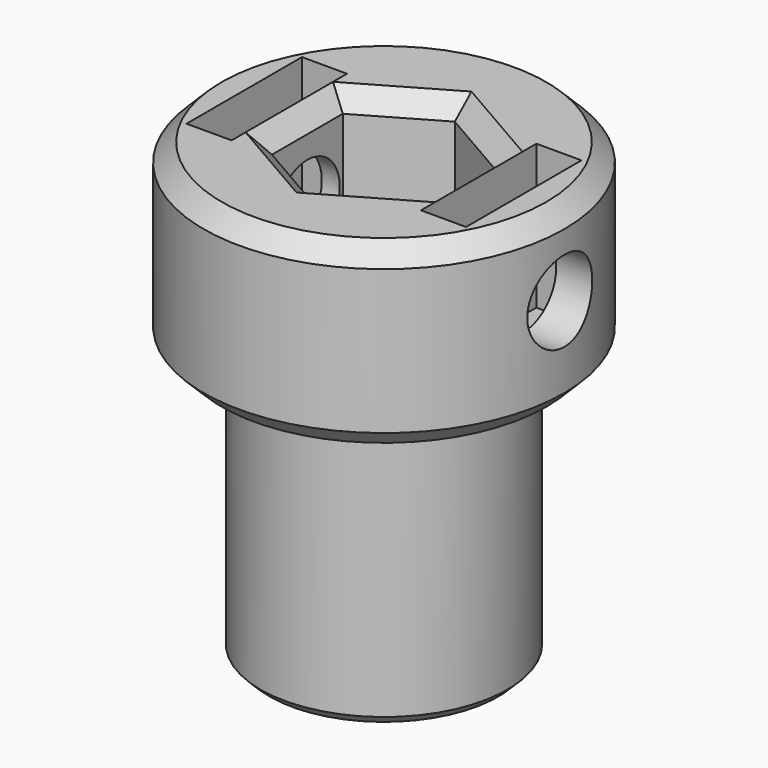
from build123d import *

# Parameters (mm, degrees)
F3_DEPTH = 25.001
F2_W     = 2.5
F2_H     = 8
F4_DEPTH = 8
F5_R     = 2.25
F6_DEPTH = 25
F7_SIZE  = 0.99999
F8_SIZE  = 0.5


# Not quite as in the source:
# - a fillet or chamfer is up to 0.001 mm smaller than in the source, because OpenCascade refuses the exact size


with BuildPart() as f1:
    # F0 (on Front) → F1 (revolve)
    with BuildSketch(Plane.XZ):
        Polygon((-6.85, 0), (0, 0), (0, 25), (-10, 25), (-10, 15), (-6.85, 15), align=None)
    revolve(axis=Axis((0, 0, 12.5), (0, 0, -1)))

    # F2 (on face) → F3 (cut, through all)
    with BuildSketch(Plane.XY.offset(25)):
        Polygon((4.25, -2.4537386441), (4.25, 2.4537386441), (0, 4.9074772881), (-4.25, 2.4537386441), (-4.25, -2.4537386441), (0, -4.9074772881), align=None)
    extrude(amount=-F3_DEPTH, mode=Mode.SUBTRACT)

    # F2 (on face) → F4 (cut)
    with BuildSketch(Plane.XY.offset(25)):
        with Locations((-6.5, 0)):
            Rectangle(F2_W, F2_H)
        with Locations((6.5, 0)):
            Rectangle(F2_W, F2_H)
    extrude(amount=-F4_DEPTH, mode=Mode.SUBTRACT)

    # F5 (on face) → F6 (cut, symmetric)
    with BuildSketch(Plane(origin=(-5.25, 0, 0), x_dir=(0, -1, 0), z_dir=(-1, 0, 0))):
        with Locations((0, 20.5)):
            Circle(F5_R)
    extrude(amount=F6_DEPTH, both=True, mode=Mode.SUBTRACT)

    # F7 (size 1 in the source; OpenCascade refuses exactly that, so slightly less here)
    f7_edges = [f1.edges().sort_by_distance(p)[0] for p in [
        (10, 0, 25),
        (10, 0, 15),
        (-2.125, 3.680608, 25),
        (2.125, 3.680608, 25),
        (4.25, 0, 25),
        (2.125, -3.680608, 25),
        (-2.125, -3.680608, 25),
        (-4.25, 0, 25),
    ]]
    chamfer(f7_edges, length=F7_SIZE)

    # F8
    f8_edges = [f1.edges().sort_by_distance(p)[0] for p in [
        (6.85, 0, 0),
        (4.25, 0, 0),
        (2.125, -3.680608, 0),
        (-2.125, -3.680608, 0),
        (-4.25, 0, 0),
        (-2.125, 3.680608, 0),
        (2.125, 3.680608, 0),
    ]]
    chamfer(f8_edges, length=F8_SIZE)


solid = f1.part
